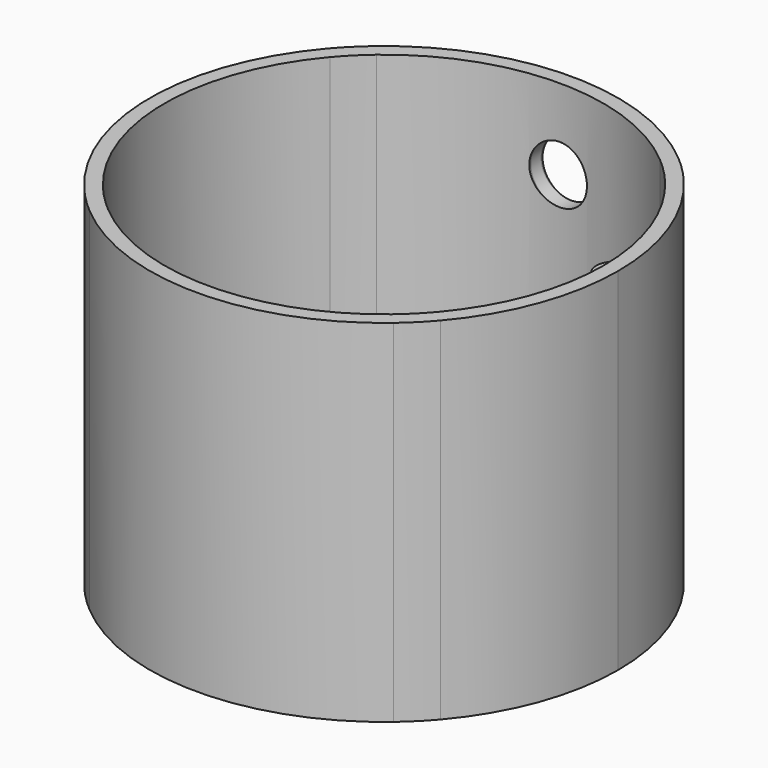
from build123d import *
from build123d import SkipClean  # not in build123d's __all__

# Parameters (mm, degrees)
F1_DEPTH = 60.96
F2_DEPTH = 45.72
F3_DEPTH = 19.05
F4_R     = 5
F5_DEPTH = 254
F6_START = -38.1
F4_R_2   = 10
F4_R_3   = 8
F4_R_4   = 7
F6_DEPTH = 2.54


with BuildPart() as f1:
    # F0 (on Top) → F1 (new body)
    with BuildSketch(Plane.XY):
        with BuildLine():
            Line((-26.4039235173, 30.8940515778), (-24.6019970286, 29.0921250892))
            ThreePointArc((-24.6019970286, 29.0921250892), (0, 38.1), (24.6019970286, 29.0921250892))
            Line((24.6019970286, 29.0921250892), (26.4039235173, 30.8940515778))
            ThreePointArc((26.4039235173, 30.8940515778), (0, 40.64), (-26.4039235173, 30.8940515778))
        make_face()
        with BuildLine():
            ThreePointArc((-24.6019970286, -29.0921250892), (-26.9407683632, -26.9407683632), (-29.0921250892, -24.6019970286))
            Line((-29.0921250892, -24.6019970286), (-30.8940515778, -26.4039235173))
            ThreePointArc((-30.8940515778, -26.4039235173), (-28.7368195874, -28.7368195874), (-26.4039235173, -30.8940515778))
            Line((-26.4039235173, -30.8940515778), (-24.6019970286, -29.0921250892))
        make_face()
        with BuildLine():
            Line((30.8940515778, 26.4039235173), (29.0921250892, 24.6019970286))
            ThreePointArc((29.0921250892, 24.6019970286), (35.7772271557, 13.0996189659), (38.1, 0))
            ThreePointArc((38.1, 0), (35.7772271557, -13.0996189659), (29.0921250892, -24.6019970286))
            Line((29.0921250892, -24.6019970286), (30.8940515778, -26.4039235173))
            ThreePointArc((30.8940515778, -26.4039235173), (38.1257383937, -14.0725858299), (40.64, 0))
            ThreePointArc((40.64, 0), (38.1257383937, 14.0725858299), (30.8940515778, 26.4039235173))
        make_face()
        with BuildLine():
            Line((26.4039235173, 30.8940515778), (24.6019970286, 29.0921250892))
            ThreePointArc((24.6019970286, 29.0921250892), (26.9407683632, 26.9407683632), (29.0921250892, 24.6019970286))
            Line((29.0921250892, 24.6019970286), (30.8940515778, 26.4039235173))
            ThreePointArc((30.8940515778, 26.4039235173), (28.7368195874, 28.7368195874), (26.4039235173, 30.8940515778))
        make_face()
        with BuildLine():
            ThreePointArc((-29.0921250892, 24.6019970286), (-26.9407683632, 26.9407683632), (-24.6019970286, 29.0921250892))
            Line((-24.6019970286, 29.0921250892), (-26.4039235173, 30.8940515778))
            ThreePointArc((-26.4039235173, 30.8940515778), (-28.7368195874, 28.7368195874), (-30.8940515778, 26.4039235173))
            Line((-30.8940515778, 26.4039235173), (-29.0921250892, 24.6019970286))
        make_face()
        with BuildLine():
            ThreePointArc((-29.0921250892, -24.6019970286), (-38.1, 0), (-29.0921250892, 24.6019970286))
            Line((-29.0921250892, 24.6019970286), (-30.8940515778, 26.4039235173))
            ThreePointArc((-30.8940515778, 26.4039235173), (-40.64, 0), (-30.8940515778, -26.4039235173))
            Line((-30.8940515778, -26.4039235173), (-29.0921250892, -24.6019970286))
        make_face()
        with BuildLine():
            ThreePointArc((24.6019970286, -29.0921250892), (0, -38.1), (-24.6019970286, -29.0921250892))
            Line((-24.6019970286, -29.0921250892), (-26.4039235173, -30.8940515778))
            ThreePointArc((-26.4039235173, -30.8940515778), (0, -40.64), (26.4039235173, -30.8940515778))
            Line((26.4039235173, -30.8940515778), (24.6019970286, -29.0921250892))
        make_face()
        with BuildLine():
            ThreePointArc((29.0921250892, -24.6019970286), (26.9407683632, -26.9407683632), (24.6019970286, -29.0921250892))
            Line((24.6019970286, -29.0921250892), (26.4039235173, -30.8940515778))
            ThreePointArc((26.4039235173, -30.8940515778), (28.7368195874, -28.7368195874), (30.8940515778, -26.4039235173))
            Line((30.8940515778, -26.4039235173), (29.0921250892, -24.6019970286))
        make_face()
    extrude(amount=F1_DEPTH)

    # F0 (on Top) → F2 (join)
    with BuildSketch(Plane.XY):
        with BuildLine():
            Line((22.225, 25.4), (20.9098719395, 25.4))
            Line((20.9098719395, 25.4), (19.9799359697, 24.4700640303))
            ThreePointArc((19.9799359697, 24.4700640303), (21.0099801022, 25.1583175157), (22.225, 25.4))
        make_face()
        with BuildLine():
            Line((25.4, 20.9098719395), (25.4, 22.225))
            ThreePointArc((25.4, 22.225), (25.1583175158, 21.0099801023), (24.4700640304, 19.9799359699))
            Line((24.4700640304, 19.9799359699), (25.4, 20.9098719395))
        make_face()
        with BuildLine():
            Line((24.6019970286, 29.0921250892), (20.9098719395, 25.4))
            Line((20.9098719395, 25.4), (22.225, 25.4))
            Line((22.225, 25.4), (25.4, 25.4))
            Line((25.4, 25.4), (25.4, 22.225))
            Line((25.4, 22.225), (25.4, 20.9098719395))
            Line((25.4, 20.9098719395), (29.0921250892, 24.6019970286))
            ThreePointArc((29.0921250892, 24.6019970286), (26.9407683632, 26.9407683632), (24.6019970286, 29.0921250892))
        make_face()
        with BuildLine():
            Line((25.4, 25.4), (22.225, 25.4))
            ThreePointArc((22.225, 25.4), (23.4400198978, 25.1583175157), (24.4700640303, 24.4700640303))
            Line((24.4700640303, 24.4700640303), (25.4, 25.4))
        make_face()
        with BuildLine():
            Line((25.4, 22.225), (25.4, 25.4))
            Line((25.4, 25.4), (24.4700640303, 24.4700640303))
            ThreePointArc((24.4700640303, 24.4700640303), (25.1583175157, 23.4400198978), (25.4, 22.225))
        make_face()
        with BuildLine():
            ThreePointArc((25.4, 22.225), (25.1583175157, 23.4400198978), (24.4700640303, 24.4700640303))
            Line((24.4700640303, 24.4700640303), (23.0242427948, 23.0242427948))
            ThreePointArc((23.0242427948, 23.0242427948), (23.2692610356, 22.6575470836), (23.3553, 22.225))
            ThreePointArc((23.3553, 22.225), (22.6575470836, 21.1807389644), (21.4257572052, 21.4257572052))
            Line((21.4257572052, 21.4257572052), (19.9799359697, 19.9799359697))
            ThreePointArc((19.9799359697, 19.9799359697), (22.2250000001, 19.05), (24.4700640304, 19.9799359699))
            ThreePointArc((24.4700640304, 19.9799359699), (25.1583175158, 21.0099801023), (25.4, 22.225))
        make_face()
        with BuildLine():
            ThreePointArc((24.4700640303, 24.4700640303), (23.4400198978, 25.1583175157), (22.225, 25.4))
            ThreePointArc((22.225, 25.4), (21.0099801022, 25.1583175157), (19.9799359697, 24.4700640303))
            ThreePointArc((19.9799359697, 24.4700640303), (19.05, 22.225), (19.9799359697, 19.9799359697))
            Line((19.9799359697, 19.9799359697), (21.4257572052, 21.4257572052))
            ThreePointArc((21.4257572052, 21.4257572052), (21.4257572052, 23.0242427948), (23.0242427948, 23.0242427948))
            Line((23.0242427948, 23.0242427948), (24.4700640303, 24.4700640303))
        make_face()
        with BuildLine():
            Line((-24.4700640303, -19.9799359697), (-25.4, -20.9098719395))
            Line((-25.4, -20.9098719395), (-25.4, -22.2250000637))
            ThreePointArc((-25.4, -22.2250000637), (-25.1583175279, -21.0099801317), (-24.4700640303, -19.9799359697))
        make_face()
        with BuildLine():
            ThreePointArc((-19.979935987, -24.4700640475), (-21.0099801135, -25.1583175204), (-22.225, -25.4))
            Line((-22.225, -25.4), (-20.9098719395, -25.4))
            Line((-20.9098719395, -25.4), (-19.979935987, -24.4700640475))
        make_face()
        with BuildLine():
            ThreePointArc((-24.4700640303, -24.4700640303), (-25.1583175035, -23.4400199272), (-25.4, -22.2250000637))
            Line((-25.4, -22.2250000637), (-25.4, -25.4))
            Line((-25.4, -25.4), (-24.4700640303, -24.4700640303))
        make_face()
        with BuildLine():
            Line((-24.4700640303, -24.4700640303), (-25.4, -25.4))
            Line((-25.4, -25.4), (-22.225, -25.4))
            ThreePointArc((-22.225, -25.4), (-23.4400198978, -25.1583175157), (-24.4700640303, -24.4700640303))
        make_face()
        with BuildLine():
            Line((-25.4, -22.2250000637), (-25.4, -20.9098719395))
            Line((-25.4, -20.9098719395), (-29.0921250892, -24.6019970286))
            ThreePointArc((-29.0921250892, -24.6019970286), (-26.9407683632, -26.9407683632), (-24.6019970286, -29.0921250892))
            Line((-24.6019970286, -29.0921250892), (-20.9098719395, -25.4))
            Line((-20.9098719395, -25.4), (-22.225, -25.4))
            Line((-22.225, -25.4), (-25.4, -25.4))
            Line((-25.4, -25.4), (-25.4, -22.2250000637))
        make_face()
        with BuildLine():
            ThreePointArc((-24.4700640303, -19.9799359697), (-25.1583175279, -21.0099801317), (-25.4, -22.2250000637))
            ThreePointArc((-25.4, -22.2250000637), (-25.1583175035, -23.4400199272), (-24.4700640303, -24.4700640303))
            Line((-24.4700640303, -24.4700640303), (-23.0242427948, -23.0242427948))
            ThreePointArc((-23.0242427948, -23.0242427948), (-23.0242427948, -21.4257572052), (-21.4257572052, -21.4257572052))
            Line((-21.4257572052, -21.4257572052), (-19.9799359697, -19.9799359697))
            ThreePointArc((-19.9799359697, -19.9799359697), (-22.225, -19.05), (-24.4700640303, -19.9799359697))
        make_face()
        with BuildLine():
            Line((-23.0242427948, -23.0242427948), (-24.4700640303, -24.4700640303))
            ThreePointArc((-24.4700640303, -24.4700640303), (-23.4400198978, -25.1583175157), (-22.225, -25.4))
            ThreePointArc((-22.225, -25.4), (-21.0099801135, -25.1583175204), (-19.979935987, -24.4700640475))
            ThreePointArc((-19.979935987, -24.4700640475), (-19.2916824889, -23.440019909), (-19.05, -22.225))
            ThreePointArc((-19.05, -22.225), (-19.2916824843, -21.0099801022), (-19.9799359697, -19.9799359697))
            Line((-19.9799359697, -19.9799359697), (-21.4257572052, -21.4257572052))
            ThreePointArc((-21.4257572052, -21.4257572052), (-21.1807389644, -21.7924529164), (-21.0947, -22.225))
            ThreePointArc((-21.0947, -22.225), (-21.7924529164, -23.2692610356), (-23.0242427948, -23.0242427948))
        make_face()
    extrude(amount=F2_DEPTH)

    # F0 (on Top) → F3 (join)
    with BuildSketch(Plane.XY):
        with BuildLine():
            Line((-20.9098719395, 25.4), (-22.225, 25.4))
            ThreePointArc((-22.225, 25.4), (-21.0099800636, 25.1583174997), (-19.9799359106, 24.4700639711))
            Line((-19.9799359106, 24.4700639711), (-20.9098719395, 25.4))
        make_face()
        with BuildLine():
            ThreePointArc((-24.4700645469, 19.9799364864), (-25.1583176555, 21.0099804398), (-25.4, 22.225))
            Line((-25.4, 22.225), (-25.4, 20.9098719395))
            Line((-25.4, 20.9098719395), (-24.4700645469, 19.9799364864))
        make_face()
        with BuildLine():
            Line((-22.225, 25.4), (-25.4, 25.4))
            Line((-25.4, 25.4), (-24.4700640303, 24.4700640303))
            ThreePointArc((-24.4700640303, 24.4700640303), (-23.4400198978, 25.1583175157), (-22.225, 25.4))
        make_face()
        with BuildLine():
            Line((-24.4700640303, 24.4700640303), (-25.4, 25.4))
            Line((-25.4, 25.4), (-25.4, 22.225))
            ThreePointArc((-25.4, 22.225), (-25.1583175157, 23.4400198978), (-24.4700640303, 24.4700640303))
        make_face()
        with BuildLine():
            ThreePointArc((-19.9799359106, 24.4700639711), (-21.0099800636, 25.1583174997), (-22.225, 25.4))
            ThreePointArc((-22.225, 25.4), (-23.4400198978, 25.1583175157), (-24.4700640303, 24.4700640303))
            Line((-24.4700640303, 24.4700640303), (-23.0242427948, 23.0242427948))
            ThreePointArc((-23.0242427948, 23.0242427948), (-21.7924529164, 23.2692610356), (-21.0947, 22.225))
            ThreePointArc((-21.0947, 22.225), (-21.1807389644, 21.7924529164), (-21.4257572052, 21.4257572052))
            Line((-21.4257572052, 21.4257572052), (-19.9799359697, 19.9799359697))
            ThreePointArc((-19.9799359697, 19.9799359697), (-19.2916824843, 21.0099801022), (-19.05, 22.225))
            ThreePointArc((-19.05, 22.225), (-19.2916824683, 23.4400198591), (-19.9799359106, 24.4700639711))
        make_face()
        with BuildLine():
            ThreePointArc((-24.4700640303, 24.4700640303), (-25.1583175157, 23.4400198978), (-25.4, 22.225))
            ThreePointArc((-25.4, 22.225), (-25.1583176555, 21.0099804398), (-24.4700645469, 19.9799364864))
            ThreePointArc((-24.4700645469, 19.9799364864), (-22.2250003653, 19.05), (-19.9799359697, 19.9799359697))
            Line((-19.9799359697, 19.9799359697), (-21.4257572052, 21.4257572052))
            ThreePointArc((-21.4257572052, 21.4257572052), (-23.0242427948, 21.4257572052), (-23.0242427948, 23.0242427948))
            Line((-23.0242427948, 23.0242427948), (-24.4700640303, 24.4700640303))
        make_face()
        with BuildLine():
            Line((-25.4, 22.225), (-25.4, 25.4))
            Line((-25.4, 25.4), (-22.225, 25.4))
            Line((-22.225, 25.4), (-20.9098719395, 25.4))
            Line((-20.9098719395, 25.4), (-24.6019970286, 29.0921250892))
            ThreePointArc((-24.6019970286, 29.0921250892), (-26.9407683632, 26.9407683632), (-29.0921250892, 24.6019970286))
            Line((-29.0921250892, 24.6019970286), (-25.4, 20.9098719395))
            Line((-25.4, 20.9098719395), (-25.4, 22.225))
        make_face()
        with BuildLine():
            Line((25.4, -20.9098719395), (24.470064035, -19.9799359744))
            ThreePointArc((24.470064035, -19.9799359744), (25.158317517, -21.0099801053), (25.4, -22.225))
            Line((25.4, -22.225), (25.4, -20.9098719395))
        make_face()
        with BuildLine():
            ThreePointArc((22.2249999363, -25.4), (21.0099802732, -25.1583175866), (19.9799362765, -24.4700643371))
            Line((19.9799362765, -24.4700643371), (20.9098719395, -25.4))
            Line((20.9098719395, -25.4), (22.2249999363, -25.4))
        make_face()
        with BuildLine():
            Line((25.4, -25.4), (25.4, -22.225))
            ThreePointArc((25.4, -22.225), (25.1583175157, -23.4400198978), (24.4700640303, -24.4700640303))
            Line((24.4700640303, -24.4700640303), (25.4, -25.4))
        make_face()
        with BuildLine():
            ThreePointArc((24.4700640303, -24.4700640303), (23.4400198683, -25.1583175279), (22.2249999363, -25.4))
            Line((22.2249999363, -25.4), (25.4, -25.4))
            Line((25.4, -25.4), (24.4700640303, -24.4700640303))
        make_face()
        with BuildLine():
            ThreePointArc((24.470064035, -19.9799359744), (22.2250000033, -19.05), (19.9799359697, -19.9799359697))
            Line((19.9799359697, -19.9799359697), (21.4257572052, -21.4257572052))
            ThreePointArc((21.4257572052, -21.4257572052), (22.6575470836, -21.1807389644), (23.3553, -22.225))
            ThreePointArc((23.3553, -22.225), (23.2692610356, -22.6575470836), (23.0242427948, -23.0242427948))
            Line((23.0242427948, -23.0242427948), (24.4700640303, -24.4700640303))
            ThreePointArc((24.4700640303, -24.4700640303), (25.1583175157, -23.4400198978), (25.4, -22.225))
            ThreePointArc((25.4, -22.225), (25.158317517, -21.0099801053), (24.470064035, -19.9799359744))
        make_face()
        with BuildLine():
            Line((21.4257572052, -21.4257572052), (19.9799359697, -19.9799359697))
            ThreePointArc((19.9799359697, -19.9799359697), (19.05, -22.2250002169), (19.9799362765, -24.4700643371))
            ThreePointArc((19.9799362765, -24.4700643371), (21.0099802732, -25.1583175866), (22.2249999363, -25.4))
            ThreePointArc((22.2249999363, -25.4), (23.4400198683, -25.1583175279), (24.4700640303, -24.4700640303))
            Line((24.4700640303, -24.4700640303), (23.0242427948, -23.0242427948))
            ThreePointArc((23.0242427948, -23.0242427948), (21.4257572052, -23.0242427948), (21.4257572052, -21.4257572052))
        make_face()
        with BuildLine():
            Line((20.9098719395, -25.4), (24.6019970286, -29.0921250892))
            ThreePointArc((24.6019970286, -29.0921250892), (26.9407683632, -26.9407683632), (29.0921250892, -24.6019970286))
            Line((29.0921250892, -24.6019970286), (25.4, -20.9098719395))
            Line((25.4, -20.9098719395), (25.4, -22.225))
            Line((25.4, -22.225), (25.4, -25.4))
            Line((25.4, -25.4), (22.2249999363, -25.4))
            Line((22.2249999363, -25.4), (20.9098719395, -25.4))
        make_face()
    extrude(amount=F3_DEPTH)

    # F4 (on Front) → F5 (cut)
    with BuildSketch(Plane.XZ):
        with Locations((0, 46.99)):
            Circle(F4_R)
    extrude(amount=-F5_DEPTH, mode=Mode.SUBTRACT)

    # F4 (on Front) → F6 (join)
    with BuildSketch(Plane.XZ.offset(F6_START)):
        with Locations((0, 46.99)):
            Circle(F4_R_2)
        with Locations((0, 46.99)):
            Circle(F4_R_3, mode=Mode.SUBTRACT)
        with Locations((0, 46.99)):
            Circle(F4_R_4)
        with Locations((0, 46.99)):
            Circle(F4_R, mode=Mode.SUBTRACT)
    with SkipClean():  # cleaning this boolean's faces spoils the solid; the shape is the same uncleaned
        extrude(amount=-F6_DEPTH)


solid = f1.part
